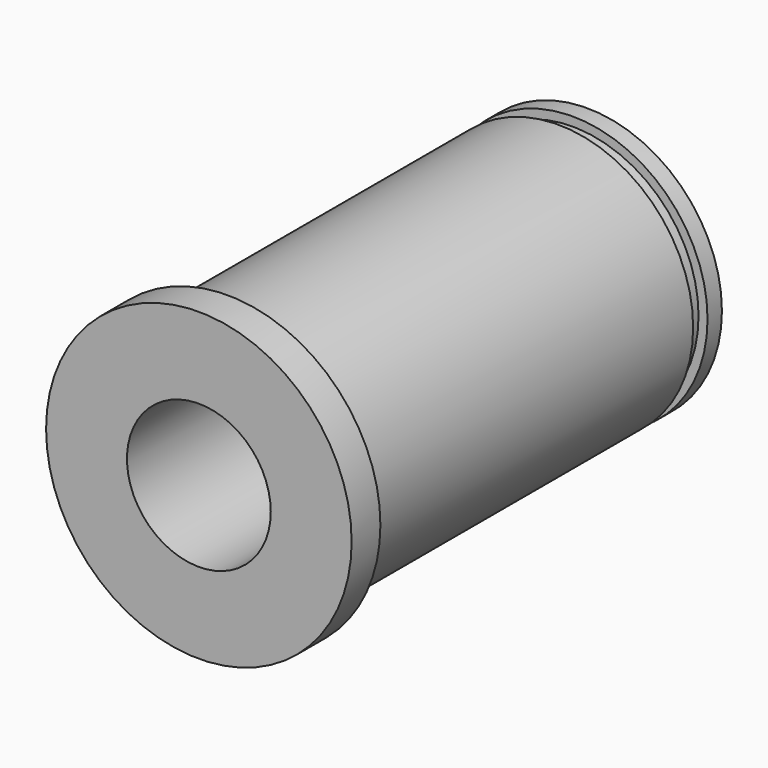
from build123d import *

# Parameters (mm, degrees)
F0_R     = 8.5
F0_R_2   = 7.5
F0_R_3   = 7
F0_R_4   = 4
F1_DEPTH = 25
F2_DEPTH = 23
F3_DEPTH = 2
F4_DEPTH = 1


with BuildPart() as f1:
    # F0 (on Front) → F1 (new body)
    with BuildSketch(Plane.XZ):
        Circle(F0_R)
        Circle(F0_R_2, mode=Mode.SUBTRACT)
        Circle(F0_R_2)
        Circle(F0_R_3, mode=Mode.SUBTRACT)
        Circle(F0_R_3)
        Circle(F0_R_4, mode=Mode.SUBTRACT)
    extrude(amount=F1_DEPTH)

    # F0 (on Front) → F2 (cut)
    with BuildSketch(Plane.XZ):
        Circle(F0_R)
        Circle(F0_R_2, mode=Mode.SUBTRACT)
    extrude(amount=F2_DEPTH, mode=Mode.SUBTRACT)

    # F0 (on Front) → F3 (join)
    with BuildSketch(Plane.XZ):
        Circle(F0_R_2)
        Circle(F0_R_3, mode=Mode.SUBTRACT)
        Circle(F0_R_3)
        Circle(F0_R_4, mode=Mode.SUBTRACT)
    extrude(amount=-F3_DEPTH)

    # F0 (on Front) → F4 (cut)
    with BuildSketch(Plane.XZ):
        Circle(F0_R_2)
        Circle(F0_R_3, mode=Mode.SUBTRACT)
    extrude(amount=-F4_DEPTH, mode=Mode.SUBTRACT)


solid = f1.part
